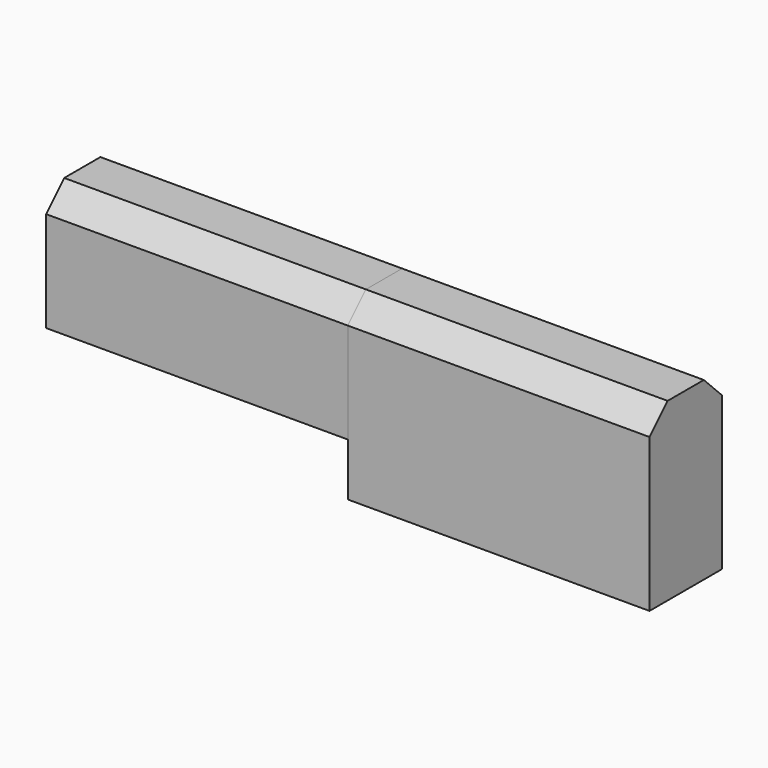
from build123d import *

# Parameters (mm, degrees)
F1_DEPTH = 40
F2_R     = 2.975
F3_DEPTH = 32
F4_SIZE  = 1
F6_DEPTH = 40
F7_R     = 3
F8_DEPTH = 32


with BuildPart() as f1:
    # F0 (on Right) → F1 (new body)
    with BuildSketch(Plane.YZ):
        Polygon((-6, 20.3), (-6, 0), (6, 0), (6, 20.3), (3, 23.3), (-3, 23.3), align=None)
    extrude(amount=F1_DEPTH)

    # F2 (on face) → F3 (join)
    with BuildSketch(Plane.YZ):
        with Locations((0, 16.8)):
            Circle(F2_R)
    extrude(amount=-F3_DEPTH)

    # F4
    f4_edges = [f1.edges().sort_by_distance(p)[0] for p in [
        (-32, -2.975, 16.8),
    ]]
    chamfer(f4_edges, length=F4_SIZE)


with BuildPart() as f6:
    # F5 (on face) → F6 (new body)
    with BuildSketch(Plane.YZ):
        Polygon((-6, 20.3), (-6, 7), (6, 7), (6, 20.3), (3, 23.3), (-3, 23.3), align=None)
    extrude(amount=-F6_DEPTH)

    # F7 (on face) → F8 (cut)
    with BuildSketch(Plane.YZ):
        with Locations((0, 16.8)):
            Circle(F7_R)
    extrude(amount=-F8_DEPTH, mode=Mode.SUBTRACT)


solid = Compound([f1.part, f6.part])
